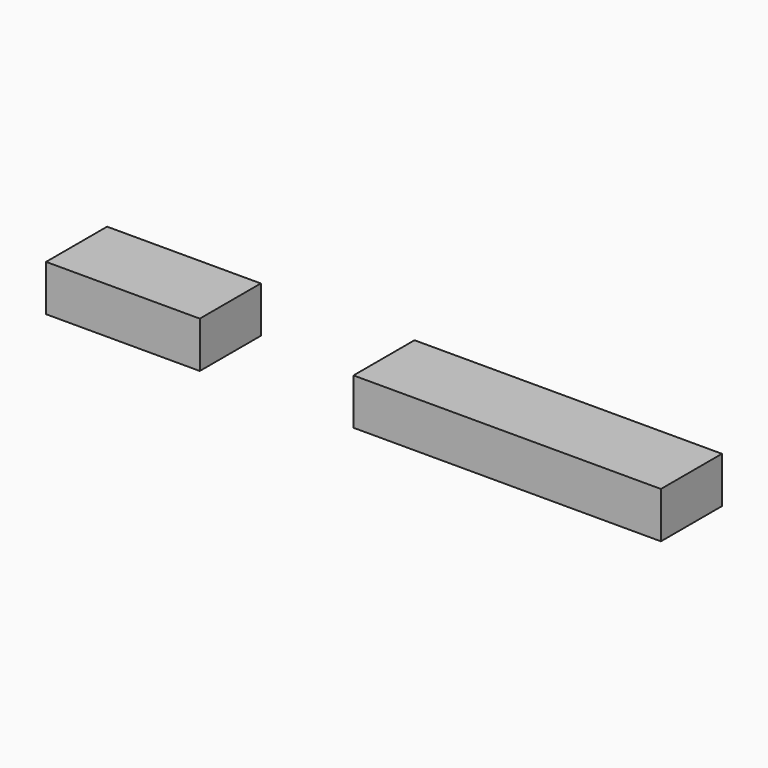
from build123d import *

# Parameters (mm, degrees)
F0_W     = 31.75
F0_H     = 9.525
F1_DEPTH = 15.748


with BuildPart() as f1:
    # F0 (on Front) → F1 (new body)
    with BuildSketch(Plane.XZ):
        with Locations((15.875, 4.7625)):
            Rectangle(F0_W, F0_H)
    extrude(amount=F1_DEPTH)


with BuildPart() as f1b:
    # F0 (on Front) → F1, piece 2 (new body)
    with BuildSketch(Plane.XZ):
        with Locations((79.375, 4.7625)):
            Rectangle(F0_W, F0_H)
        with Locations((111.125, 4.7625)):
            Rectangle(F0_W, F0_H)
    extrude(amount=F1_DEPTH)


solid = Compound([f1.part, f1b.part])
